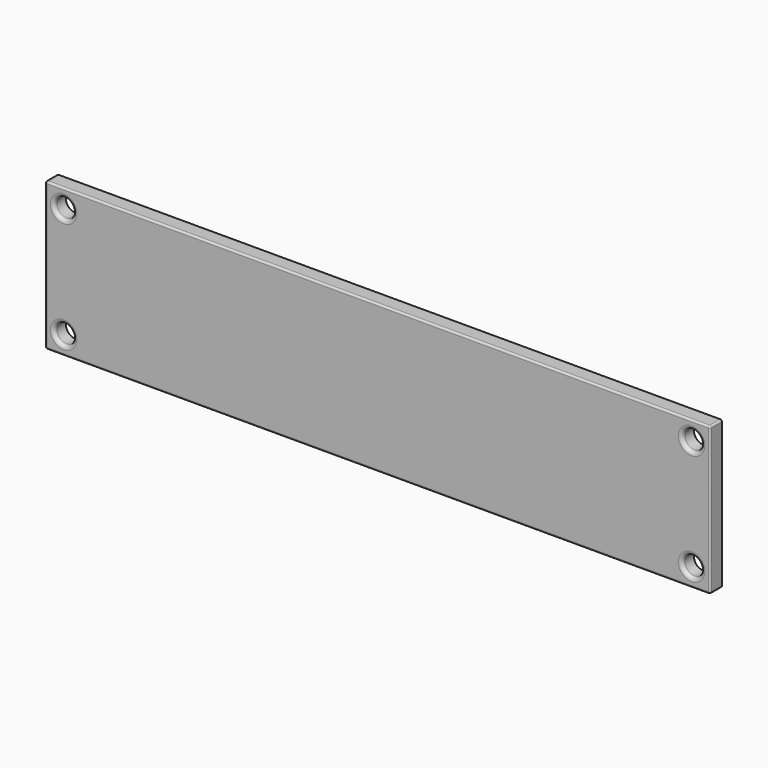
from build123d import *

# Parameters (mm, degrees)
F0_W         = 180
F0_H         = 40
F0_R         = 2.5751263091
F1_DEPTH     = 4
F2_R         = 1
F3_R         = 0.5
F4_TEXT_SIZE = 12.1815817022
F5_DEPTH     = 1


# Not quite as in the source:
# - a feature names something its author has since deleted; it is built from what else it names
# - Text() gives the source's letters only with a copy of the font that has no kerning and outlines rounded to 1/6400 em; it was checked with that copy


with BuildPart() as f1:
    # F0 (on Front) → F1 (new body)
    with BuildSketch(Plane.XZ):
        Rectangle(F0_W, F0_H)
        with Locations((-85, -15)):
            Circle(F0_R, mode=Mode.SUBTRACT)
        with Locations((85, -15)):
            Circle(F0_R, mode=Mode.SUBTRACT)
        with Locations((-85, 15)):
            Circle(F0_R, mode=Mode.SUBTRACT)
        with Locations((85, 15)):
            Circle(F0_R, mode=Mode.SUBTRACT)
    extrude(amount=F1_DEPTH)

    # F2
    f2_edges = [f1.edges().sort_by_distance(p)[0] for p in [
        (-87.575126, -4, 15),
        (-87.575126, -4, -15),
        (82.424874, -4, 15),
        (82.424874, -4, -15),
    ]]
    fillet(f2_edges, radius=F2_R)

    # F3
    f3_edges = [f1.edges().sort_by_distance(p)[0] for p in [
        (0, -4, 20),
        (-90, -4, 0),
        (0, -4, -20),
        (90, -4, 0),
        (-90, -2, 20),
        (-90, -2, -20),
        (90, -2, 20),
        (90, -2, -20),
    ]]
    fillet(f3_edges, radius=F3_R)

    # F4 (on face) → F5 (join)
    with BuildSketch(Plane(origin=(0, 0, 0), x_dir=(-1, 0, 0), z_dir=(0, 1, 0))):
        with Locations((-64.9919360876, -2.0154650365)):
            Text('Virage Cap', F4_TEXT_SIZE, font='Open Sans', text_align=(TextAlign.LEFT, TextAlign.BOTTOM))
    extrude(amount=F5_DEPTH)

    # F6: F1 across plane


with BuildPart() as f1_1:
    add(f1.part)
    add(f1.part.mirror(Plane.YZ))


solid = f1_1.part
